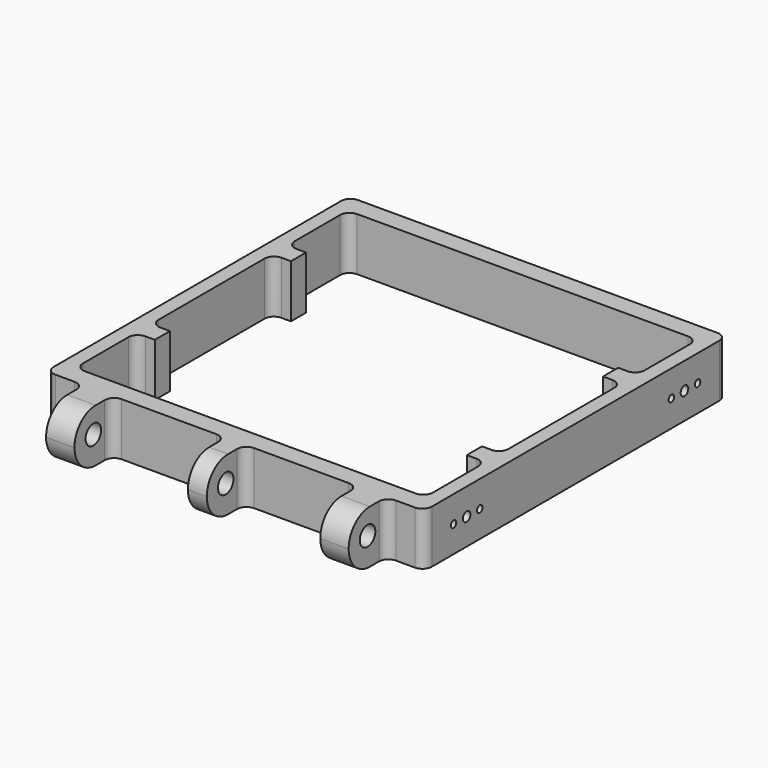
from build123d import *

# Parameters (mm, degrees)
F0_W      = 9.525
F0_H      = 15.875
F0_W_2    = 6.35
F1_DEPTH  = 17.78
F3_DEPTH  = 17.781
F4_R      = 3.175
F7_R      = 3.2639
F8_DEPTH  = 114.301
F9_R      = 8.89
F10_R     = 8.88999
F11_R     = 1.5875
F11_R_2   = 1.143
F12_DEPTH = 3.175
F15_R     = 1.5875
F15_R_2   = 1.143
F16_DEPTH = 3.175


# Not quite as in the source:
# - two fillets or chamfers of one size are made in one step
# - a fillet or chamfer is up to 0.001 mm smaller than in the source, because OpenCascade refuses the exact size


with BuildPart() as f1:
    # F0 (on Top) → F1 (new body)
    with BuildSketch(Plane.XY):
        Polygon((63.5, 57.15), (-63.5, 57.15), (-63.5, -69.85), (-50.8, -69.85), (-41.275, -69.85), (-3.175, -69.85), (3.175, -69.85), (41.275, -69.85), (50.8, -69.85), (63.5, -69.85), align=None)
        with Locations((-46.0375, -77.7875)):
            Rectangle(F0_W, F0_H)
        with Locations((46.0375, -77.7875)):
            Rectangle(F0_W, F0_H)
        with Locations((0, -77.7875)):
            Rectangle(F0_W_2, F0_H)
    extrude(amount=F1_DEPTH)

    # F2 (on face) → F3 (cut, through all)
    with BuildSketch(Plane.XY.offset(17.78)):
        Polygon((3.175, 50.8), (-58.7375, 50.8), (-58.7375, 25.4), (-52.3875, 25.4), (-52.3875, 19.05), (-58.7375, 19.05), (-58.7375, -31.75), (-52.3875, -31.75), (-52.3875, -38.1), (-58.7375, -38.1), (-58.7375, -63.5), (3.175, -63.5), (58.7375, -63.5), (58.7375, -38.1), (52.3875, -38.1), (52.3875, -31.75), (58.7375, -31.75), (58.7375, 19.05), (52.3875, 19.05), (52.3875, 25.4), (58.7375, 25.4), (58.7375, 50.8), align=None)
    extrude(amount=-F3_DEPTH, mode=Mode.SUBTRACT)

    # F4
    f4_edges = [f1.edges().sort_by_distance(p)[0] for p in [
        (-58.7375, 50.8, 8.89),
        (63.5, 57.15, 8.89),
        (-63.5, 57.15, 8.89),
        (63.5, -69.85, 8.89),
        (-63.5, -69.85, 8.89),
        (50.8, -69.85, 8.89),
        (-50.8, -69.85, 8.89),
        (41.275, -69.85, 8.89),
        (-41.275, -69.85, 8.89),
        (3.175, -69.85, 8.89),
        (-3.175, -69.85, 8.89),
        (58.7375, 25.4, 8.89),
        (58.7375, 50.8, 8.89),
        (-58.7375, 25.4, 8.89),
        (-58.7375, 19.05, 8.89),
        (-58.7375, -31.75, 8.89),
        (-58.7375, -38.1, 8.89),
        (-58.7375, -63.5, 8.89),
        (58.7375, -63.5, 8.89),
        (58.7375, -38.1, 8.89),
        (58.7375, -31.75, 8.89),
        (58.7375, 19.05, 8.89),
    ]]
    fillet(f4_edges, radius=F4_R)

    # F7 (on face) → F8 (cut, through all)
    with BuildSketch(Plane(origin=(-50.8, 0, 0), x_dir=(0, -1, 0), z_dir=(-1, 0, 0))):
        with Locations((77.7875, 9.525)):
            Circle(F7_R)
    extrude(amount=-F8_DEPTH, mode=Mode.SUBTRACT)

    # F9
    f9_edges = [f1.edges().sort_by_distance(p)[0] for p in [
        (-46.0375, -85.725, 17.78),
        (0, -85.725, 17.78),
        (46.0375, -85.725, 17.78),
    ]]
    fillet(f9_edges, radius=F9_R)

    # F10 (radius 8.89 in the source; OpenCascade refuses exactly that, so slightly less here)
    f10_edges = [f1.edges().sort_by_distance(p)[0] for p in [
        (-46.0375, -85.725, 0),
        (0, -85.725, 0),
        (46.0375, -85.725, 0),
    ]]
    fillet(f10_edges, radius=F10_R)

    # F11 (on face) → F12 (cut)
    with BuildSketch(Plane.YZ.offset(63.5)):
        with Locations((-52.07, 8.89)):
            Circle(F11_R)
        with Locations((-46.5709, 8.89)):
            Circle(F11_R_2)
        with Locations((39.37, 8.89)):
            Circle(F11_R)
        with Locations((33.8709, 8.89)):
            Circle(F11_R_2)
        with Locations((-57.5691, 8.89)):
            Circle(F11_R_2)
        with Locations((44.8691, 8.89)):
            Circle(F11_R_2)
    extrude(amount=-F12_DEPTH, mode=Mode.SUBTRACT)

    # F15 (on face) → F16 (cut)
    with BuildSketch(Plane(origin=(-63.5, 0, 0), x_dir=(0, -1, 0), z_dir=(-1, 0, 0))):
        with Locations((-39.37, 8.89)):
            Circle(F15_R)
        with Locations((-33.8709, 8.89)):
            Circle(F15_R_2)
        with Locations((-44.8691, 8.89)):
            Circle(F15_R_2)
        with Locations((52.07, 8.89)):
            Circle(F15_R)
        with Locations((57.5691, 8.89)):
            Circle(F15_R_2)
        with Locations((46.5709, 8.89)):
            Circle(F15_R_2)
    extrude(amount=-F16_DEPTH, mode=Mode.SUBTRACT)


solid = f1.part
